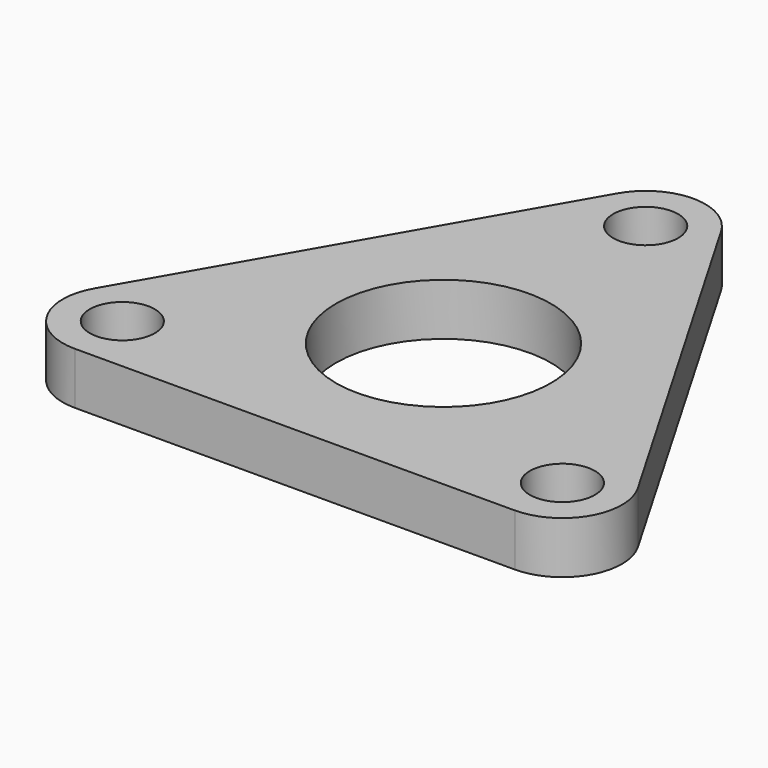
from build123d import *

# Parameters (mm, degrees)
F1_DEPTH = 5.08
F2_D     = 21
F3_D     = 6.35
F4_D     = 6.35
F5_D     = 6.35


with BuildPart() as f1:
    # F0 (on Top) → F1 (new body)
    with BuildSketch(Plane.XY):
        with BuildLine():
            Line((26.5037064396, -9.4034548087), (4.9663911618, 27.6804330928))
            ThreePointArc((4.9663911618, 27.6804330928), (-0.0783700027, 30.5758122309), (-5.1082224721, 27.6546104755))
            Line((-5.1082224721, 27.6546104755), (-26.455153827, -9.5391956352))
            ThreePointArc((-26.455153827, -9.5391956352), (-26.440245132, -15.3557765287), (-21.3954839675, -18.2511556668))
            Line((-21.3954839675, -18.2511556668), (21.4887626653, -18.1412374576))
            ThreePointArc((21.4887626653, -18.1412374576), (26.5186151347, -15.2200357022), (26.5037064396, -9.4034548087))
        make_face()
    extrude(amount=F1_DEPTH)

    # F2 (through all)
    with Locations(Plane(origin=(0, 0, 0), x_dir=(1, 0, 0), z_dir=(0, 0, -1))):
        with Locations((0, 0)):
            Hole(F2_D / 2)

    # F3 (through all)
    with Locations(Plane(origin=(0, 0, 0), x_dir=(1, 0, 0), z_dir=(0, 0, -1))):
        with Locations((-21.4103926626, 12.4345747733)):
            Hole(F3_D / 2)

    # F4 (through all)
    with Locations(Plane(origin=(0, 0, 0), x_dir=(1, 0, 0), z_dir=(0, 0, -1))):
        with Locations((21.4738539702, 12.3246565641)):
            Hole(F4_D / 2)

    # F5 (through all)
    with Locations(Plane(origin=(0, 0, 0), x_dir=(1, 0, 0), z_dir=(0, 0, -1))):
        with Locations((-0.0634613077, -24.7592313374)):
            Hole(F5_D / 2)


solid = f1.part
